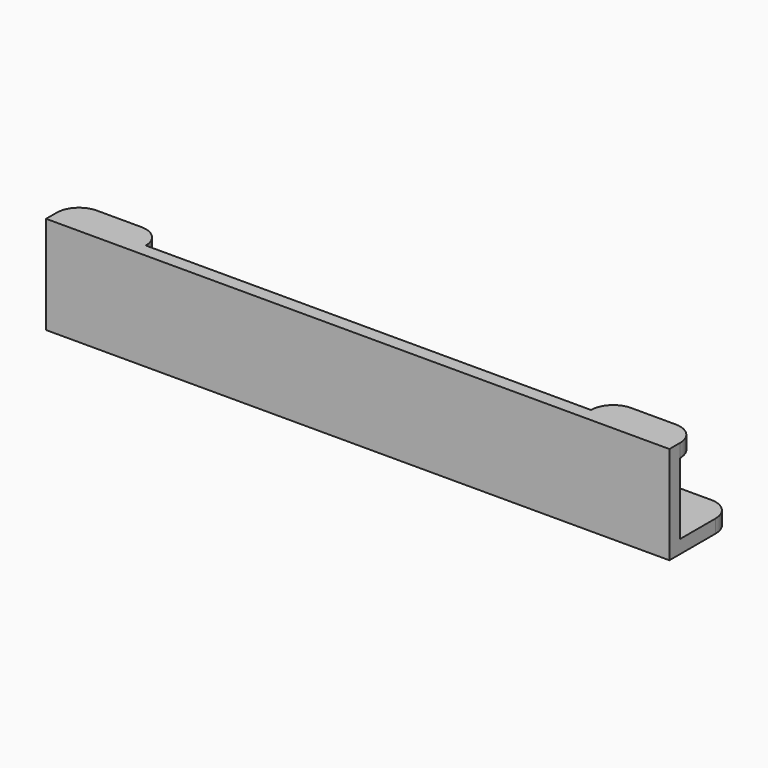
from build123d import *

# Parameters (mm, degrees)
F0_W         = 140
F0_H         = 22
F1_DEPTH     = 3
F2_W         = 140
F2_H         = 3
F3_DEPTH     = 15
F2_W_2       = 20
F4_DEPTH     = 5
F5_R         = 4.99999
F6_TEXT_SIZE = 12.026232219
F7_DEPTH     = 1


# Not quite as in the source:
# - a fillet or chamfer is up to 0.001 mm smaller than in the source, because OpenCascade refuses the exact size
# - Text() gives the source's letters only with a copy of the font that has no kerning and outlines rounded to 1/6400 em; it was checked with that copy


with BuildPart() as f1:
    # F0 (on Front) → F1 (new body)
    with BuildSketch(Plane.XZ):
        with Locations((0, 11)):
            Rectangle(F0_W, F0_H)
    extrude(amount=F1_DEPTH)

    # F2 (on face) → F3 (join)
    with BuildSketch(Plane(origin=(0, 0, 0), x_dir=(-1, 0, 0), z_dir=(0, 1, 0))):
        with Locations((0, 1.5)):
            Rectangle(F2_W, F2_H)
    extrude(amount=F3_DEPTH)

    # F2 (on face) → F4 (join)
    with BuildSketch(Plane(origin=(0, 0, 0), x_dir=(-1, 0, 0), z_dir=(0, 1, 0))):
        with Locations((60, 20.5)):
            Rectangle(F2_W_2, F2_H)
        with Locations((-60, 20.5)):
            Rectangle(F2_W_2, F2_H)
    extrude(amount=F4_DEPTH)

    # F5 (radius 5 in the source; OpenCascade refuses exactly that, so slightly less here)
    f5_edges = [f1.edges().sort_by_distance(p)[0] for p in [
        (-70, 15, 1.5),
        (70, 15, 1.5),
        (70, 5, 20.5),
        (50, 5, 20.5),
        (-70, 5, 20.5),
        (-50, 5, 20.5),
    ]]
    fillet(f5_edges, radius=F5_R)

    # F6 (on face) → F7 (cut)
    with BuildSketch(Plane(origin=(0, 0, 0), x_dir=(-1, 0, 0), z_dir=(0, 1, 0))):
        with Locations(Location((50, 16), (0, 0, 180))):
            Text('Dybbol3Dprint.dk', F6_TEXT_SIZE, font='Open Sans', text_align=(TextAlign.LEFT, TextAlign.BOTTOM))
    extrude(amount=-F7_DEPTH, mode=Mode.SUBTRACT)


solid = f1.part
